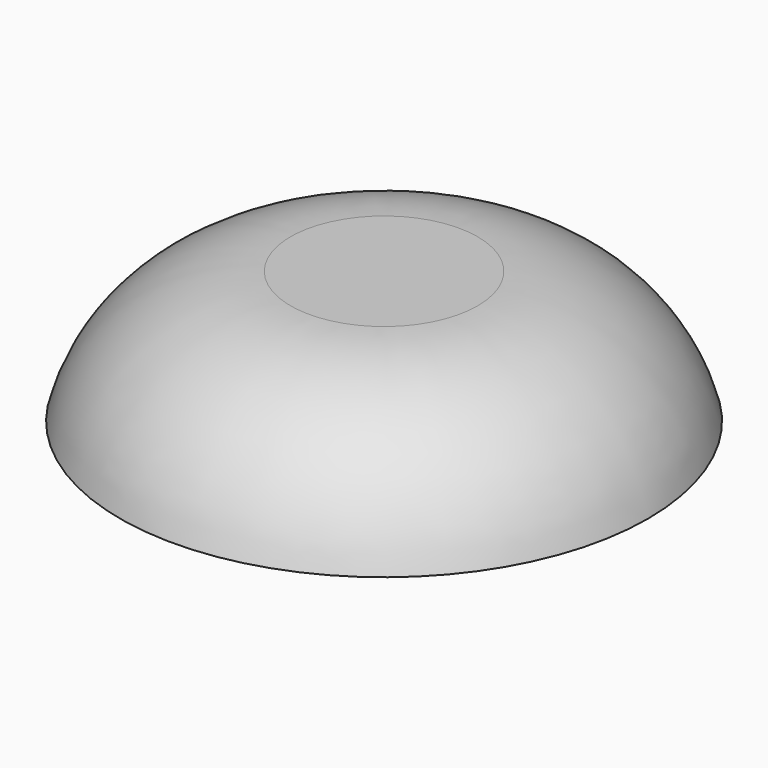
from build123d import *

# Parameters (mm, degrees)
F0_R     = 7.62
F1_DEPTH = 3.81
F3_R     = 5.715
F4_DEPTH = 1.27


# Not quite as in the source:
# - a fillet or chamfer that OpenCascade refuses, or shapes differently, is made with other operations: its cross-section is extruded or revolved along the edge and cut away or added


with BuildPart() as f1:
    # F0 (on Top) → F1 (new body)
    with BuildSketch(Plane.XY):
        Circle(F0_R)
    extrude(amount=F1_DEPTH)

    # F2: fillet of radius 5.08 on 1 edges, made by hand

    # F2_s1 → F2_t2 (revolve, cut)
    with BuildSketch(Plane.XZ):
        with BuildLine():
            ThreePointArc((7.62, 0), (5.8121631237, 2.7460926284), (2.7013111503, 3.81))
            Line((2.7013111503, 3.81), (7.62, 3.81))
            Line((7.62, 3.81), (7.62, 0))
        make_face()
    revolve(axis=Axis((0, 0, 3.81), (0, 0, 1)), mode=Mode.SUBTRACT)

    # F3 (on face) → F4 (cut)
    with BuildSketch(Plane(origin=(0, 0, 0), x_dir=(1, 0, 0), z_dir=(0, 0, -1))):
        Circle(F3_R)
    extrude(amount=-F4_DEPTH, mode=Mode.SUBTRACT)


solid = f1.part
